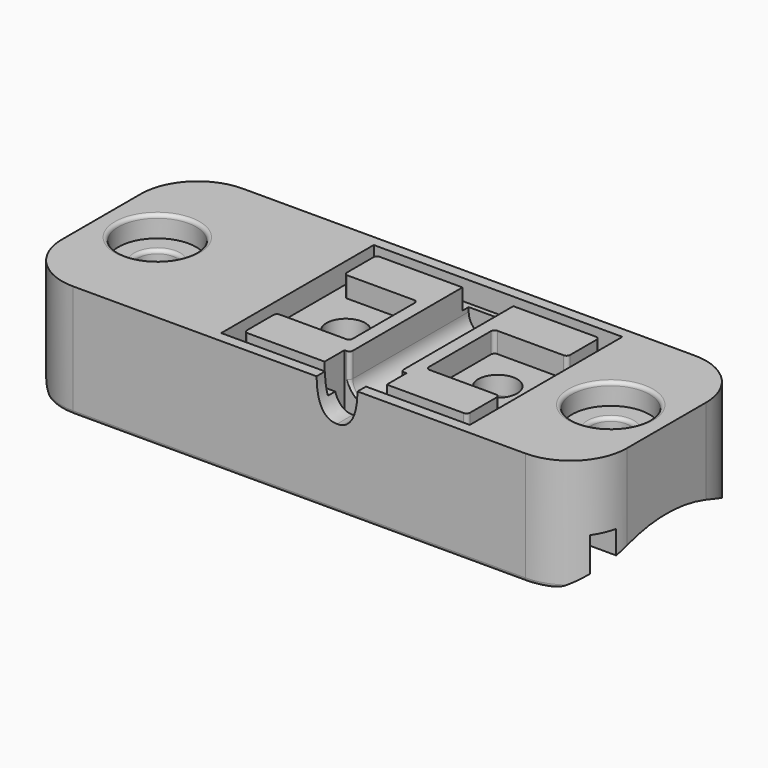
from build123d import *

# Parameters (mm, degrees)
F0_R          = 2.75
F1_DEPTH      = 14
F2_R          = 22.5
F3_DEPTH      = 45
F4_R          = 5.5
F4_R_2        = 2.75
F5_DEPTH      = 1
F6_R          = 5.5
F7_DEPTH      = 10
F8_W          = 7.2
F8_H          = 21
F8_W_2        = 0.8
F8_H_2        = 4
F9_DEPTH      = 4
F11_DEPTH     = 2
F13_R         = 0.5
F15_DEPTH     = 2.8
F16_DEPTH     = 14.0010001
F18_DEPTH     = 34.5
F19_T1_DEPTH  = 20.5
F19_T6_ANGLE  = 359.64
F19_T11_ANGLE = 359.64
F20_R         = 2.75
F21_DEPTH     = 2.9
F22_R         = 0.5
F23_R         = 0.3


# Not quite as in the source:
# - a fillet or chamfer that OpenCascade refuses, or shapes differently, is made with other operations: its cross-section is extruded or revolved along the edge and cut away or added
# - a feature names something its author has since deleted; it is built from what else it names


with BuildPart() as f1:
    # F0 (on Top) → F1 (new body)
    with BuildSketch(Plane.XY):
        with BuildLine():
            Line((-32, -15), (0, -15))
            Line((0, -15), (32, -15))
            ThreePointArc((32, -15), (37.6568542495, -12.6568542495), (40, -7))
            Line((40, -7), (40, 7))
            ThreePointArc((40, 7), (37.6568542495, 12.6568542495), (32, 15))
            Line((32, 15), (0, 15))
            Line((0, 15), (-32, 15))
            ThreePointArc((-32, 15), (-37.6568542495, 12.6568542495), (-40, 7))
            Line((-40, 7), (-40, -7))
            ThreePointArc((-40, -7), (-37.6568542495, -12.6568542495), (-32, -15))
        make_face()
        with Locations((-32.1, 0)):
            Circle(F0_R, mode=Mode.SUBTRACT)
        with Locations((-5.4, 0)):
            Circle(F0_R, mode=Mode.SUBTRACT)
        with Locations((16.1, 0)):
            Circle(F0_R, mode=Mode.SUBTRACT)
        with Locations((32.1, 0)):
            Circle(F0_R, mode=Mode.SUBTRACT)
    extrude(amount=F1_DEPTH)

    # F2 (on Right) → F3 (cut, symmetric)
    with BuildSketch(Plane.YZ):
        with Locations((0, -17.5)):
            Circle(F2_R)
    extrude(amount=F3_DEPTH, both=True, mode=Mode.SUBTRACT)

    # F4 (on face) → F5 (cut)
    with BuildSketch(Plane.XY.offset(14)):
        with Locations((32.1, 0)):
            Circle(F4_R)
        with Locations((32.1, 0)):
            Circle(F4_R_2, mode=Mode.SUBTRACT)
        with Locations((-32.1, 0)):
            Circle(F4_R)
        with Locations((-32.1, 0)):
            Circle(F4_R_2, mode=Mode.SUBTRACT)
    extrude(amount=-F5_DEPTH, mode=Mode.SUBTRACT)

    # F6 (on face) → F7 (cut)
    with BuildSketch(Plane.XY):
        Polygon((19.1711153401, 5.1961524227), (13.1711153401, 5.1961524227), (10.1711153401, 0), (13.1711153401, -5.1961524227), (19.1711153401, -5.1961524227), (22.1711153401, 0), align=None)
        Polygon((-8.4, -5.1961524227), (-2.4, -5.1961524227), (0.6, 0), (-2.4, 5.1961524227), (-8.4, 5.1961524227), (-11.4, 0), align=None)
        with Locations((-32.1, 0)):
            Circle(F6_R)
        with Locations((32.1, 0)):
            Circle(F6_R)
    extrude(amount=F7_DEPTH, mode=Mode.SUBTRACT)

    # F8 (on face) → F9 (cut)
    with BuildSketch(Plane.XY.offset(14)):
        with Locations((5.35, 2.3)):
            Rectangle(F8_W, F8_H)
        with Locations((1.35, -10.2)):
            Rectangle(F8_W_2, F8_H_2)
        Polygon((1.75, -8.2), (1.75, -12.2), (2.55, -12.2), (8.15, -12.2), (8.95, -12.2), (8.95, -8.2), align=None)
        with Locations((9.35, -10.2)):
            Rectangle(F8_W_2, F8_H_2)
    extrude(amount=-F9_DEPTH, mode=Mode.SUBTRACT)

    # F11 (add): faces of the model
    f11_faces = [f1.faces().sort_by_distance(p)[0] for p in [
        (-0.6514327417, 0.0058717003, 14),
        (-0.6514327417, 0.0058717003, 14),
    ]]
    extrude(f11_faces, amount=F11_DEPTH)

    # F13
    f13_edges = [f1.edges().sort_by_distance(p)[0] for p in [
        (1.75, -8.2, 13),
        (8.95, -8.2, 13),
        (26.6, 0, 16),
        (-37.6, 0, 16),
        (-34.85, 0, 13),
        (29.35, 0, 13),
        (-34.85, 0, 10),
        (-8.15, 0, 10),
        (13.35, 0, 10),
        (29.35, 0, 10),
        (0, 15, 0),
        (0, -15, 0),
    ]]
    fillet(f13_edges, radius=F13_R)

    # F14 (on face) → F15 (cut, through all)
    with BuildSketch(Plane.XZ.offset(15)):
        with BuildLine():
            Line((8.25, 16), (5.35, 16))
            Line((5.35, 16), (2.45, 16))
            add(Edge.make_bspline(
                [(2.45, 16), (2.4636389963, 13.8166910037), (2.9653143138, 10.9900690839), (5.35, 11)],
                knots=[0, 0, 0, 0, 5.7801384066, 5.7801384066, 5.7801384066, 5.7801384066], degree=3))
            add(Edge.make_bspline(
                [(8.25, 16), (8.2363610037, 13.8166910037), (7.7346856862, 10.9900690839), (5.35, 11)],
                knots=[0, 0, 0, 0, 5.7801384066, 5.7801384066, 5.7801384066, 5.7801384066], degree=3))
        make_face()
    extrude(amount=-F15_DEPTH, mode=Mode.SUBTRACT)

    # F8 (on face) → F16 (cut, through all)
    with BuildSketch(Plane.XY.offset(14)):
        Polygon((1.75, -8.2), (1.75, -12.2), (2.55, -12.2), (8.15, -12.2), (8.95, -12.2), (8.95, -8.2), align=None)
        with Locations((1.35, -10.2)):
            Rectangle(F8_W_2, F8_H_2)
        with Locations((9.35, -10.2)):
            Rectangle(F8_W_2, F8_H_2)
    extrude(amount=-F16_DEPTH, mode=Mode.SUBTRACT)

    # F17 (on face) → F18 (cut)
    with BuildSketch(Plane.YZ.offset(40)):
        Polygon((-8.6836605117, 0), (-8.6836605117, 6.5744962582), (-11.6836605117, 6.5744962582), (-11.6836605117, 3.8834047803), (-11.6836605117, 0), align=None)
    extrude(amount=-F18_DEPTH, mode=Mode.SUBTRACT)

    # F19: fillet of radius 2.5 on 2 edges, made by hand

    # F19_s2 → F19_t1 (join)
    with BuildSketch(Plane.XZ.offset(-12.8)):
        with BuildLine():
            ThreePointArc((8.95, 12.5), (8.217766953, 10.732233047), (6.45, 10))
            Line((6.45, 10), (8.95, 10))
            Line((8.95, 10), (8.95, 12.5))
        make_face()
        with BuildLine():
            ThreePointArc((1.75, 12.5), (2.482233047, 10.732233047), (4.25, 10))
            Line((4.25, 10), (1.75, 10))
            Line((1.75, 10), (1.75, 12.5))
        make_face()
    extrude(amount=F19_T1_DEPTH)


with BuildPart() as f19_tool4:
    # F19_s5 → F19_t6 (revolve)
    with BuildSketch(Plane(origin=(0.0484286009, -7.7075497951, 0), x_dir=(0, 0, 1), z_dir=(0.006283144, -0.9999802609, 0))):
        with BuildLine():
            ThreePointArc((12.5, -1.7015951175), (10.732233047, -2.4338281646), (10, -4.2015951175))
            Line((10, -4.2015951175), (10, -1.7015951175))
            Line((10, -1.7015951175), (12.5, -1.7015951175))
        make_face()
    revolve(axis=Axis((1.25, -7.7, 10), (0, 0, 1)), revolution_arc=F19_T6_ANGLE)

    split(bisect_by=Plane.XZ.offset(8.2), keep=Keep.BOTTOM)


with BuildPart() as f1_1:
    add(f1.part)

    # F19_t3: union F19_tool4
    add(f19_tool4.part)


with BuildPart() as f19_tool9:
    # F19_s10 → F19_t11 (revolve)
    with BuildSketch(Plane.XZ.offset(7.7)):
        with BuildLine():
            ThreePointArc((8.95, 12.5), (8.217766953, 10.732233047), (6.45, 10))
            Line((6.45, 10), (8.95, 10))
            Line((8.95, 10), (8.95, 12.5))
        make_face()
    revolve(axis=Axis((9.45, -7.7, 10), (0, 0, 1)), revolution_arc=F19_T11_ANGLE)

    split(bisect_by=Plane.XZ.offset(8.2), keep=Keep.BOTTOM)


with BuildPart() as f1_2:
    add(f1_1.part)

    # F19_t8: union F19_tool9
    add(f19_tool9.part)

    # F20 (on face) → F21 (cut)
    with BuildSketch(Plane.XY.offset(16)):
        Polygon((5.35, 13.5), (-12.25, 13.5), (-12.25, -13.5), (2.45, -13.5), (2.45, -12.2), (0.95, -12.2), (0.95, -11.7), (-10.45, -11.7), (-10.45, -6), (-0.05, -6), (-0.05, 6), (-10.45, 6), (-10.45, 11.7), (1.75, 11.7), (1.75, 12.8), (5.35, 12.8), align=None)
        with Locations((-5.4, 0)):
            Circle(F20_R, mode=Mode.SUBTRACT)
        Polygon((22.95, 13.5), (5.35, 13.5), (5.35, 12.8), (8.95, 12.8), (8.95, 11.7), (21.15, 11.7), (21.15, 6), (10.75, 6), (10.75, -6), (21.15, -6), (21.15, -11.7), (9.75, -11.7), (9.75, -12.2), (8.25, -12.2), (8.25, -13.5), (22.95, -13.5), align=None)
        with Locations((16.1, 0)):
            Circle(F20_R, mode=Mode.SUBTRACT)
        Polygon((2.45, -12.2), (2.45, -13.5), (5.35, -13.5), (5.35, -11.7), (0.95, -11.7), (0.95, -12.2), align=None)
        Polygon((5.35, -11.7), (5.35, -13.5), (8.25, -13.5), (8.25, -12.2), (9.75, -12.2), (9.75, -11.7), align=None)
    extrude(amount=-F21_DEPTH, mode=Mode.SUBTRACT)

    # F22
    f22_edges = [f1_2.edges().sort_by_distance(p)[0] for p in [
        (-0.05, 6, 14.55),
        (-10.45, 6, 14.55),
        (-10.45, 11.7, 14.55),
        (21.15, 6, 14.55),
        (-10.45, -6, 14.55),
        (-10.45, -11.7, 14.55),
        (21.15, -11.7, 14.55),
        (-0.05, -6, 14.55),
        (10.75, -6, 14.55),
        (21.15, -6, 14.55),
        (10.75, 6, 14.55),
        (21.15, 11.7, 14.55),
    ]]
    fillet(f22_edges, radius=F22_R)

    # F23
    f23_edges = [f1_2.edges().sort_by_distance(p)[0] for p in [
        (-9.892287, 2.611436, 4.84794),
        (-9.892287, -2.611436, 4.84794),
        (-5.4, -5.196152, 4.391779),
        (-0.907713, -2.611436, 4.84794),
        (-0.907713, 2.611436, 4.84794),
        (-5.4, 5.196152, 4.391779),
        (16.171115, 5.196152, 4.391779),
        (11.678829, 2.611436, 4.84794),
        (11.678829, -2.611436, 4.84794),
        (16.171115, -5.196152, 4.391779),
        (20.663402, -2.611436, 4.84794),
        (20.663402, 2.611436, 4.84794),
        (-37.599997, 0.005441, 4.999999),
        (26.600003, 0.005441, 4.999999),
    ]]
    fillet(f23_edges, radius=F23_R)


solid = f1_2.part
